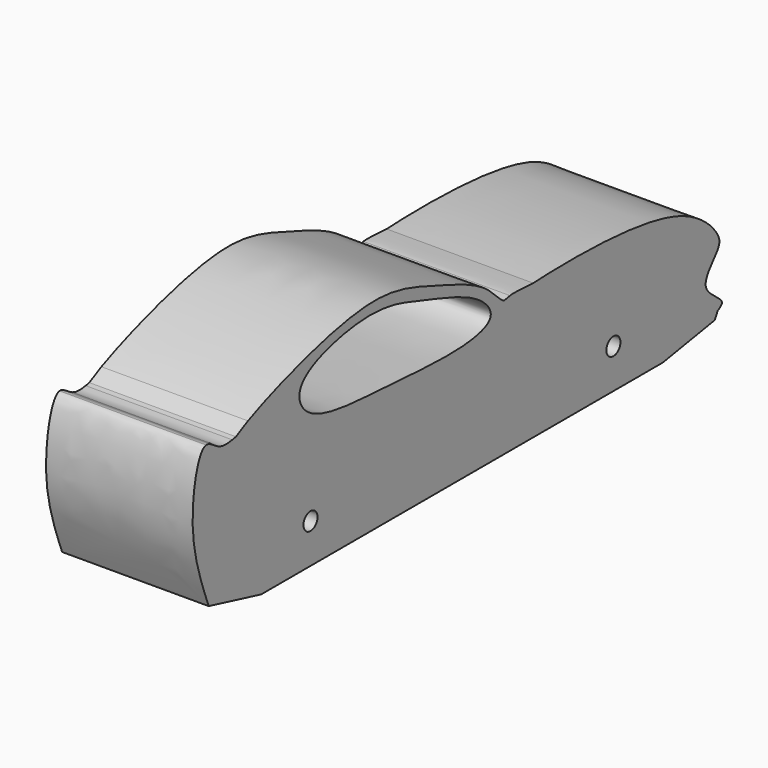
from build123d import *

# Parameters (mm, degrees)
F0_R     = 1.5
F1_DEPTH = 25


# Not quite as in the source:
# - ends of sketch curves that miss each other by under 0.0002 mm in the source are joined


with BuildPart() as f1:
    # F0 (on Right) → F1 (new body)
    with BuildSketch(Plane.YZ):
        with BuildLine():
            Line((-50.7617667317, -3.9528077468), (-39.5860101343, -6.7379684187))
            Line((-39.5860101343, -6.7379684187), (46.0432308973, -6.7379684187))
            Line((46.0432308973, -6.7379684187), (57.1172684431, -4.8679746687))
            Line((57.1172684431, -4.8679746687), (57.7666796744, -3.6975014955))
            add(Edge.make_bspline(
                [(57.7666796744, -3.6975014955), (57.9269304735, -3.6154532476), (58.2733235693, -3.4381003312), (59.3799558366, -2.3965590054), (52.7882713216, 0.7631539546), (58.3659024563, 5.3860688493), (58.0571974107, 8.1266536165), (49.7599488602, 16.5839839353), (23.9790894249, 16.7151150187), (19.7543554778, 16.4872427397), (18.4364598244, 16.4161585271)],
                knots=[0, 0, 0, 0, 0.0421262894, 0.0910588644, 0.2129396027, 0.3379442497, 0.4185309664, 0.5963044285, 0.8740681317, 1, 1, 1, 1], degree=3))
            add(Edge.make_bspline(
                [(18.4364598244, 16.4161585271), (16.2206014954, 16.5693663982), (14.0047431663, 16.7225742692), (13.4836259445, 16.5483725941)],
                knots=[0, 0, 0, 0, 0.0655694392, 0.0655694392, 0.0655694392, 0.0655694392], degree=3))
            add(Edge.make_bspline(
                [(13.4836259445, 16.5483725941), (13.3873086229, 16.5161751574), (13.2466334708, 16.3573400952), (14.7474277587, 15.7089670563), (13.1069939562, 15.7604147816), (12.2113176019, 16.2666239703), (11.9916052565, 16.4161585271)],
                knots=[0.0655694392, 0.0655694392, 0.0655694392, 0.0655694392, 0.0776885412, 0.1099409897, 0.1510702344, 0.1647232953, 0.1647232953, 0.1647232953, 0.1647232953], degree=3))
            add(Edge.make_bspline(
                [(11.9916052565, 16.4161585271), (10.8881838132, 17.1671387969), (8.0810417065, 20.8751520927), (-3.6561887816, 24.835855888), (-16.2589625009, 29.8781421357), (-36.1311443469, 23.2714548953), (-42.3939600587, 20.4621553421)],
                knots=[0.1647232953, 0.1647232953, 0.1647232953, 0.1647232953, 0.2332905856, 0.3543845074, 0.4843473591, 0.6624081206, 0.6624081206, 0.6624081206, 0.6624081206], degree=3))
            add(Edge.make_bspline(
                [(-42.3939600587, 20.4621553421), (-43.6608214877, 19.7981957582), (-44.9434164115, 19.1259902806), (-44.9606844562, 19.126215279), (-44.9608363738, 19.126249876)],
                knots=[0, 0, 0, 0, 0.9822017525, 0.9943999818, 0.9943999818, 0.9943999818, 0.9943999818], degree=3))
            add(Edge.make_bspline(
                [(-44.9608363738, 19.126249876), (-45.2207392187, 19.0744983362), (-45.4806396185, 19.0227575334), (-45.7397623572, 18.9780683416)],
                knots=[0, 0, 0, 0, 0.0374796446, 0.0374796446, 0.0374796446, 0.0374796446], degree=3))
            add(Edge.make_bspline(
                [(-45.7397623572, 18.9780683416), (-46.9233606978, 18.5463747034), (-47.8139149927, 18.4740200675), (-48.5388413072, 19.1263109446)],
                knots=[0.7002673095, 0.7002673095, 0.7002673095, 0.7002673095, 0.7490371773, 0.7490371773, 0.7490371773, 0.7490371773], degree=3))
            add(Edge.make_bspline(
                [(-48.5388413072, 19.1263109446), (-49.5471573808, 19.5561542116), (-50.4925358438, 20.5566980211), (-51.3253266106, 20.4552034955)],
                knots=[0.1758530505, 0.1758530505, 0.1758530505, 0.1758530505, 0.3315134752, 0.3315134752, 0.3315134752, 0.3315134752], degree=3))
            add(Edge.make_bspline(
                [(-51.3253266106, 20.4552034955), (-51.561234628, 15.9902543964), (-51.1615006799, 6.0187233248), (-50.7617667317, -3.9528077468)],
                knots=[0.8697497195, 0.8697497195, 0.8697497195, 0.8697497195, 1, 1, 1, 1], degree=3))
        make_face()
        with Locations((-29.0574878454, 0)):
            Circle(F0_R, mode=Mode.SUBTRACT)
        with Locations((35.5147086084, 0)):
            Circle(F0_R, mode=Mode.SUBTRACT)
        with BuildLine():
            add(Edge.make_bspline(
                [(9.3358792365, 15.1179311797), (9.0440196202, 14.0497210886), (3.4835189443, 12.3345448267), (-13.2205234696, 13.7992261366), (-29.8516494715, 14.3598370966), (-33.2641992094, 22.7984772466), (-17.2585013037, 26.7713148109), (-8.8300077425, 24.713242527), (-4.152979197, 22.9849053285), (6.5076164708, 19.8743526848), (9.6154167418, 16.1410421807), (9.3358792365, 15.1179311797)],
                knots=[0, 0, 0, 0, 0.0827339246, 0.2394822314, 0.3867125696, 0.46785692, 0.6054276443, 0.7150666011, 0.7973013084, 0.9207590444, 1, 1, 1, 1], degree=3))
        make_face(mode=Mode.SUBTRACT)
        with BuildLine():
            add(Edge.make_bspline(
                [(-51.3253266106, 20.4552034955), (-51.3875377964, 20.4476216454), (-53.0480696079, 20.0773587702), (-55.5823777844, 8.6739953508), (-52.4528517495, 0.4767131805), (-50.7617667317, -3.9528077468)],
                knots=[0.3315134752, 0.3315134752, 0.3315134752, 0.3315134752, 0.3431416296, 0.6450570034, 1, 1, 1, 1], degree=3))
            add(Edge.make_bspline(
                [(-51.3253266083, 20.455203495), (-51.561234628, 15.9902543964), (-51.1615006799, 6.0187233248), (-50.7617667317, -3.9528077468)],
                knots=[0.8697497195, 0.8697497195, 0.8697497195, 0.8697497195, 1, 1, 1, 1], degree=3))
        make_face()
        with BuildLine():
            add(Edge.make_bspline(
                [(-45.7397623572, 18.9780683416), (-46.6964335383, 18.8130775653), (-47.6425047492, 18.7442043368), (-48.5388413072, 19.1263109446)],
                knots=[0.0374796446, 0.0374796446, 0.0374796446, 0.0374796446, 0.1758530505, 0.1758530505, 0.1758530505, 0.1758530505], degree=3))
            add(Edge.make_bspline(
                [(-45.7397623572, 18.9780683416), (-46.9233606978, 18.5463747034), (-47.8139149927, 18.4740200675), (-48.5388413072, 19.1263109446)],
                knots=[0.7002673095, 0.7002673095, 0.7002673095, 0.7002673095, 0.7490371773, 0.7490371773, 0.7490371773, 0.7490371773], degree=3))
        make_face()
        with BuildLine():
            add(Edge.make_bspline(
                [(13.4836259445, 16.5483725941), (13.3873086229, 16.5161751574), (13.2466334708, 16.3573400952), (14.7474277587, 15.7089670563), (13.1069939562, 15.7604147816), (12.2113176019, 16.2666239703), (11.9916052565, 16.4161585271)],
                knots=[0.0655694392, 0.0655694392, 0.0655694392, 0.0655694392, 0.0776885412, 0.1099409897, 0.1510702344, 0.1647232953, 0.1647232953, 0.1647232953, 0.1647232953], degree=3))
            add(Edge.make_bspline(
                [(13.4836259445, 16.5483725941), (13.2742123616, 16.5175567669), (12.8681111875, 16.4577977796), (12.3067005276, 16.3081530164), (12.0859181381, 16.3838308095), (11.9916052565, 16.4161585271)],
                knots=[0, 0, 0, 0, 0.3788383409, 0.7346548055, 1, 1, 1, 1], degree=3))
        make_face()
    extrude(amount=F1_DEPTH)


solid = f1.part
